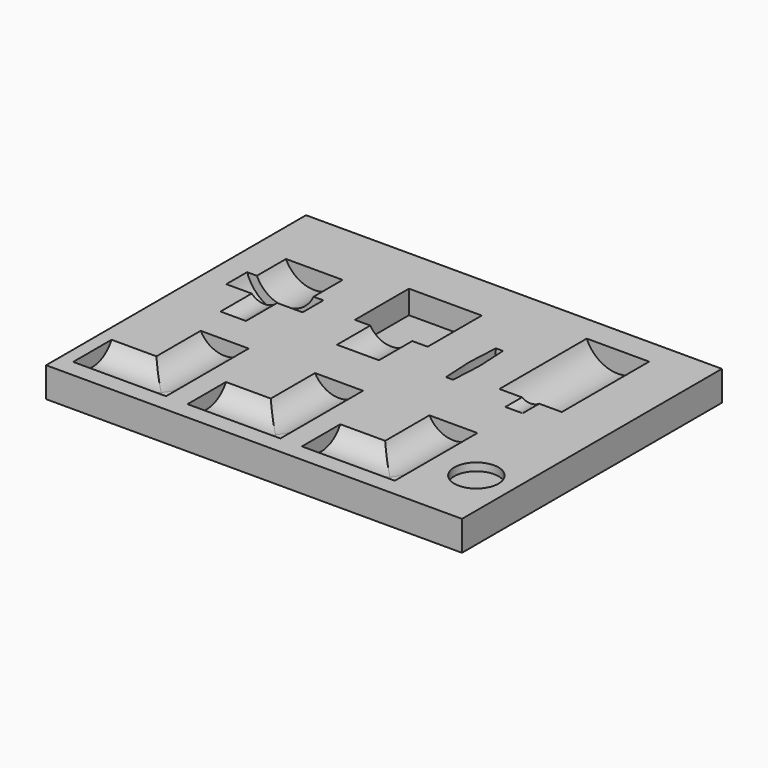
from build123d import *

# Parameters (mm, degrees)
F0_W      = 160
F0_H      = 125
F1_DEPTH  = 16.5
F2_W      = 37
F2_H      = 10.5
F4_W      = 10.5
F4_H      = 41
F6_W      = 10.5
F6_H      = 41
F8_W      = 10.5
F8_H      = 41
F10_R     = 8.5
F11_DEPTH = 8
F14_W     = 9.5
F14_H     = 16
F17_DEPTH = 14
F20_W     = 160
F20_H     = 5
F21_DEPTH = 150
F24_W     = 18.4661853126
F24_H     = 1.2669073437
F24_W_2   = 1.2669073437
F24_H_2   = 18.4661853126
F25_DEPTH = 10
F27_START = -10.5
F27_DEPTH = 1


with BuildPart() as f1:
    # F0 (on Top) → F1 (new body)
    with BuildSketch(Plane.XY):
        with Locations((80, 62.5)):
            Rectangle(F0_W, F0_H)
    extrude(amount=-F1_DEPTH)

    # F2 (on face) → F3 (revolve, cut)
    with BuildSketch(Plane.XY):
        with Locations((23.5, 10.75)):
            Rectangle(F2_W, F2_H)
        with Locations((67.5, 10.75)):
            Rectangle(F2_W, F2_H)
        with Locations((111.5, 10.75)):
            Rectangle(F2_W, F2_H)
    revolve(axis=Axis((23.5, 16, 0), (1, 0, 0)), mode=Mode.SUBTRACT)

    # F4 (on face) → F5 (revolve, cut)
    with BuildSketch(Plane.XY):
        with Locations((36.75, 26)):
            Rectangle(F4_W, F4_H)
    revolve(axis=Axis((31.5, 26, 0), (0, 1, 0)), mode=Mode.SUBTRACT)

    # F6 (on face) → F7 (revolve, cut)
    with BuildSketch(Plane.XY):
        with Locations((80.75, 26)):
            Rectangle(F6_W, F6_H)
    revolve(axis=Axis((75.5, 26, 0), (0, 1, 0)), mode=Mode.SUBTRACT)

    # F8 (on face) → F9 (revolve, cut)
    with BuildSketch(Plane.XY):
        with Locations((124.75, 26)):
            Rectangle(F8_W, F8_H)
    revolve(axis=Axis((119.5, 26, 0), (0, 1, 0)), mode=Mode.SUBTRACT)

    # F10 (on face) → F11 (cut)
    with BuildSketch(Plane.XY):
        with Locations((145.7579010625, 24.7283919918)):
            Circle(F10_R)
    extrude(amount=-F11_DEPTH, mode=Mode.SUBTRACT)

    # F12 (on face) → F13 (revolve, cut)
    with BuildSketch(Plane.XY):
        Polygon((24, 75), (24, 60), (31, 60), (31, 75), (39.5, 75), (39.5, 85), (36, 85), (36, 99), (28.5, 99), (28.5, 113), (24, 113), (24, 99), (24, 85), align=None)
    revolve(axis=Axis((24, 92, 0), (0, 1, 0)), mode=Mode.SUBTRACT)

    # F14 (on face) → F15 (revolve, cut)
    with BuildSketch(Plane.XY):
        with Locations((72.75, 73)):
            Rectangle(F14_W, F14_H)
    revolve(axis=Axis((68, 73, 0), (0, 1, 0)), mode=Mode.SUBTRACT)

    # F16 (on face) → F17 (cut)
    with BuildSketch(Plane.XY):
        Polygon((54, 107), (54, 81), (58.5, 81), (77.5, 81), (82, 81), (82, 107), align=None)
    extrude(amount=-F17_DEPTH, mode=Mode.SUBTRACT)

    # F18 (on face) → F19 (revolve, cut)
    with BuildSketch(Plane.XY):
        Polygon((128, 73), (128, 65), (134, 65), (134, 73), (141, 73), (141, 115), (128, 115), align=None)
    revolve(axis=Axis((128, 94, 0), (0, 1, 0)), mode=Mode.SUBTRACT)

    # F20 (on Front) → F21 (cut)
    with BuildSketch(Plane.XZ):
        with Locations((80, -2.5)):
            Rectangle(F20_W, F20_H)
    extrude(amount=-F21_DEPTH, mode=Mode.SUBTRACT)

    # F22 (on face) → F23 (revolve, cut)
    with BuildSketch(Plane.XY.offset(-5)):
        Polygon((98.6288933514, 93), (98, 81), (102, 81), (101.3711066486, 93), align=None)
    revolve(axis=Axis((100, 81, -5), (1, 0, 0)), mode=Mode.SUBTRACT)

    # F24 (on face) → F25 (join)
    with BuildSketch(Plane.XY.offset(-5)):
        with Locations((31.5, 6.1334536718)):
            Rectangle(F24_W, F24_H)
        with Locations((41.3665463282, 16)):
            Rectangle(F24_W_2, F24_H_2)
        with Locations((85.3665463282, 16)):
            Rectangle(F24_W_2, F24_H_2)
        with Locations((75.5, 6.1334536718)):
            Rectangle(F24_W, F24_H)
        with Locations((129.3665463282, 16)):
            Rectangle(F24_W_2, F24_H_2)
        with Locations((119.5, 6.1334536718)):
            Rectangle(F24_W, F24_H)
    extrude(amount=-F25_DEPTH)

    # F26 (on face) → F27 (join)
    with BuildSketch(Plane.XY.offset(-5).offset(F27_START)):
        Polygon((101.528329799, 90.0000035763), (98.471670201, 90.0000035763), (98, 81), (98.3558213304, 74.210524559), (101.6441786696, 74.210524559), (102, 81), align=None)
    extrude(amount=-F27_DEPTH)


solid = f1.part
